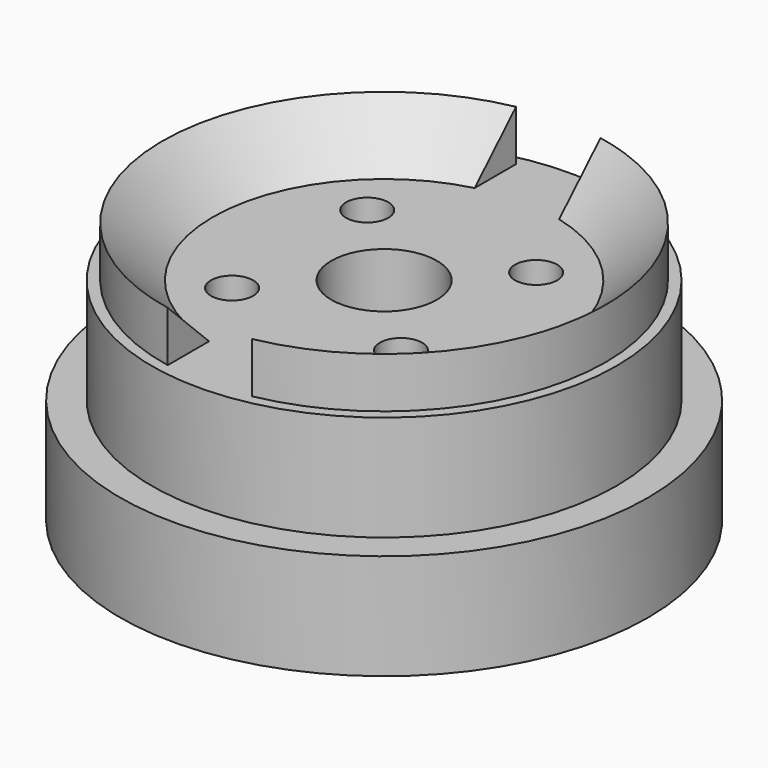
from build123d import *

# Parameters (mm, degrees)
F0_R        = 12.5
F0_R_2      = 11
F1_DEPTH    = 5
F0_R_3      = 1
F2_DEPTH    = 10
F3_DEPTH    = 15
F4_T4_ANGLE = 333.3635987438
F4_T9_ANGLE = 333.3635987438
F5_D        = 5
F5_DEPTH    = 12
F5_TIP      = 1.5021515476
F6_DEPTH    = 8


# Not quite as in the source:
# - a fillet or chamfer that OpenCascade refuses, or shapes differently, is made with other operations: its cross-section is extruded or revolved along the edge and cut away or added


with BuildPart() as f1:
    # F0 (on Top) → F1 (new body)
    with BuildSketch(Plane.XY):
        Circle(F0_R)
        Circle(F0_R_2, mode=Mode.SUBTRACT)
    extrude(amount=F1_DEPTH)

    # F0 (on Top) → F2 (join)
    with BuildSketch(Plane.XY):
        Circle(F0_R_2)
        with Locations((-4, -4)):
            Circle(F0_R_3, mode=Mode.SUBTRACT)
        with Locations((4, -4)):
            Circle(F0_R_3, mode=Mode.SUBTRACT)
        with BuildLine():
            ThreePointArc((-2, -10.307764064), (-10.5, 0), (-2, 10.307764064))
            Line((-2, 10.307764064), (-2, 7.8581159461))
            ThreePointArc((-2, 7.8581159461), (-8.1086365206, 0), (-2, -7.8581159461))
            Line((-2, -7.8581159461), (-2, -10.307764064))
        make_face(mode=Mode.SUBTRACT)
        with Locations((-4, 4)):
            Circle(F0_R_3, mode=Mode.SUBTRACT)
        with Locations((4, 4)):
            Circle(F0_R_3, mode=Mode.SUBTRACT)
        with BuildLine():
            ThreePointArc((2, 10.307764064), (10.5, 0), (2, -10.307764064))
            Line((2, -10.307764064), (2, -7.8581159461))
            ThreePointArc((2, -7.8581159461), (8.1086365206, 0), (2, 7.8581159461))
            Line((2, 7.8581159461), (2, 10.307764064))
        make_face(mode=Mode.SUBTRACT)
    extrude(amount=F2_DEPTH)

    # F0 (on Top) → F3 (join)
    with BuildSketch(Plane.XY):
        with BuildLine():
            Line((-2, 7.8581159461), (-2, 10.307764064))
            ThreePointArc((-2, 10.307764064), (-10.5, 0), (-2, -10.307764064))
            Line((-2, -10.307764064), (-2, -7.8581159461))
            ThreePointArc((-2, -7.8581159461), (-8.1086365206, 0), (-2, 7.8581159461))
        make_face()
        with BuildLine():
            Line((2, -7.8581159461), (2, -10.307764064))
            ThreePointArc((2, -10.307764064), (10.5, 0), (2, 10.307764064))
            Line((2, 10.307764064), (2, 7.8581159461))
            ThreePointArc((2, 7.8581159461), (8.1086365206, 0), (2, -7.8581159461))
        make_face()
    extrude(amount=F3_DEPTH)

    # F4: chamfer of 5 on 2 edges, made by hand


with BuildPart() as f4_tool2:
    # F4_s3 → F4_t4 (revolve)
    with BuildSketch(Plane(origin=(0, 0, 0), x_dir=(0, 0, 1), z_dir=(0.2303588664, 0.9731057459, 0))):
        Polygon((10, 8.1086365206), (15, 13.1086365206), (15, 8.1086365206), align=None)
    revolve(axis=Axis((0, 0, 15), (0, 0, -1)), revolution_arc=F4_T4_ANGLE)

    split(bisect_by=Plane.XY.offset(10), keep=Keep.TOP)


with BuildPart() as f1_1:
    add(f1.part)

    # F4_t1: cut F4_tool2
    add(f4_tool2.part, mode=Mode.SUBTRACT)


with BuildPart() as f4_tool7:
    # F4_s8 → F4_t9 (revolve)
    with BuildSketch(Plane(origin=(0, 0, 0), x_dir=(0, 0, 1), z_dir=(-0.2303588664, -0.9731057459, 0))):
        Polygon((10, 8.1086365206), (15, 13.1086365206), (15, 8.1086365206), align=None)
    revolve(axis=Axis((0, 0, 15), (0, 0, -1)), revolution_arc=F4_T9_ANGLE)

    split(bisect_by=Plane.XY.offset(10), keep=Keep.TOP)


with BuildPart() as f1_2:
    add(f1_1.part)

    # F4_t6: cut F4_tool7
    add(f4_tool7.part, mode=Mode.SUBTRACT)

    # F5
    with Locations(Plane(origin=(0, 0, 0), x_dir=(1, 0, 0), z_dir=(0, 0, -1))):
        with Locations((0, 0)):
            Hole(F5_D / 2, depth=F5_DEPTH)
            with Locations((0, 0, -(F5_DEPTH + F5_TIP / 2))):  # 118° drill point
                Cone(0, F5_D / 2, F5_TIP, mode=Mode.SUBTRACT)

    # F0 (on Top) → F6 (join)
    with BuildSketch(Plane.XY):
        with Locations((-4, 4)):
            Circle(F0_R_3)
        with Locations((4, 4)):
            Circle(F0_R_3)
        with Locations((-4, -4)):
            Circle(F0_R_3)
        with Locations((4, -4)):
            Circle(F0_R_3)
    extrude(amount=F6_DEPTH)


solid = f1_2.part
